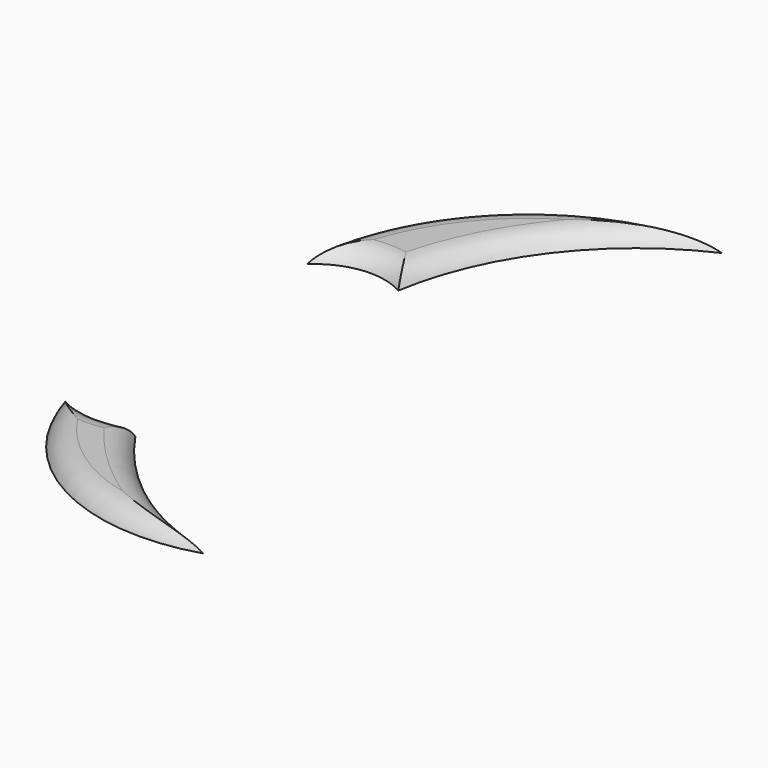
from build123d import *

# Parameters (mm, degrees)
F4_DEPTH      = 3
F5_T2_ANGLE   = 62.2477049864
F5_T4_ANGLE   = 129.1340791789
F5_T6_ANGLE   = 126.4050370347
F5_2_T2_ANGLE = 80.8778277447
F5_2_T4_ANGLE = 111.257856834
F5_2_T6_ANGLE = 169.7853810378


# Not quite as in the source:
# - a fillet or chamfer that OpenCascade refuses, or shapes differently, is made with other operations: its cross-section is extruded or revolved along the edge and cut away or added
# - a feature of the source that left no trace in its solid (it failed there, or was rolled back) is left out
# - the program builds the solid bodies; features that only make, move or delete a surface that nothing else refers to are left out


with BuildPart() as f4:
    # F3 (on Top) → F4 (new body)
    with BuildSketch(Plane.XY):
        with BuildLine():
            ThreePointArc((-5.3077070042, -31.2650799751), (-13.2021361292, -31.9649934775), (-20.5774232745, -29.0637817234))
            ThreePointArc((-20.5774232745, -29.0637817234), (-2.4043363453, -51.7875856508), (26.5503625851, -54.6612180769))
            ThreePointArc((26.5503625851, -54.6612180769), (8.5747716437, -45.7499050222), (-5.3077070042, -31.2650799751))
        make_face()
    extrude(amount=F4_DEPTH)

    # F5: fillet of radius 5 on 3 edges, made by hand

    # F5_s1 → F5_t2 (revolve, cut)
    with BuildSketch(Plane(origin=(42.5768459914, -3.8517260252, 0), x_dir=(0, 0, 1), z_dir=(0.9959329635, -0.0900973481, 0))):
        with BuildLine():
            ThreePointArc((0, 53.1706891683), (2.1833001327, 55.0146520758), (3, 57.7532648633))
            Line((3, 57.7532648633), (3, 53.1706891683))
            Line((3, 53.1706891683), (0, 53.1706891683))
        make_face()
    revolve(axis=Axis((43.0309999283, 1.1684758534, 3), (0, 0, -1)), revolution_arc=F5_T2_ANGLE, mode=Mode.SUBTRACT)

    # F5_s3 → F5_t4 (revolve, cut)
    with BuildSketch(Plane(origin=(-10.1562466974, -15.2654101251, 0), x_dir=(0, 0, 1), z_dir=(0.5539186056, 0.8325708248, 0))):
        with BuildLine():
            ThreePointArc((0, 16.5640855704), (2.1833001327, 18.4080484779), (3, 21.1466612654))
            Line((3, 21.1466612654), (3, 16.5640855704))
            Line((3, 16.5640855704), (0, 16.5640855704))
        make_face()
    revolve(axis=Axis((-10.7388300445, -14.8778109616, 3), (0, 0, -1)), revolution_arc=F5_T4_ANGLE, mode=Mode.SUBTRACT)

    # F5_s5 → F5_t6 (revolve, cut)
    with BuildSketch(Plane(origin=(-0.548879568, -18.3736765408, 0), x_dir=(0, 0, 1), z_dir=(0.029859828, 0.9995540959, 0))):
        with BuildLine():
            ThreePointArc((0, -21.4392018096), (2.1833001327, -19.5952389021), (3, -16.8566261146))
            Line((3, -16.8566261146), (3, -21.4392018096))
            Line((3, -21.4392018096), (0, -21.4392018096))
        make_face()
    revolve(axis=Axis((15.4842666098, -18.8526370977, 3), (0, 0, 1)), revolution_arc=F5_T6_ANGLE, mode=Mode.SUBTRACT)


with BuildPart() as f4b:
    # F3 (on Top) → F4, piece 2 (new body)
    with BuildSketch(Plane.XY):
        with BuildLine():
            ThreePointArc((-4.1721854359, 30.9002492577), (6.0474831917, 54.8040980412), (26.3369232416, 71.057535708))
            ThreePointArc((26.3369232416, 71.057535708), (-4.9982200607, 58.9572788508), (-20.3394051641, 29.0749184787))
            ThreePointArc((-20.3394051641, 29.0749184787), (-12.5583392109, 32.6672592136), (-4.1721854359, 30.9002492577))
        make_face()
    extrude(amount=F4_DEPTH)

    # F5#2: fillet of radius 5 on 3 edges, made by hand

    # F5_2_s1 → F5_2_t2 (revolve, cut)
    with BuildSketch(Plane(origin=(-1.1051572436, 19.683889291, 0), x_dir=(0, 0, 1), z_dir=(0.0560569838, -0.998427571, 0))):
        with BuildLine():
            ThreePointArc((0, 3.6571197259), (2.1833001327, 5.5010826334), (3, 8.2396954209))
            Line((3, 8.2396954209), (3, 3.6571197259))
            Line((3, 3.6571197259), (0, 3.6571197259))
        make_face()
    revolve(axis=Axis((48.6007815653, 22.4746425569, 3), (0, 0, -1)), revolution_arc=F5_2_T2_ANGLE, mode=Mode.SUBTRACT)

    # F5_2_s3 → F5_2_t4 (revolve, cut)
    with BuildSketch(Plane(origin=(19.5896273479, -4.7607351825, 0), x_dir=(0, 0, 1), z_dir=(0.9717166727, -0.2361497577, 0))):
        with BuildLine():
            ThreePointArc((0, -76.6524312792), (2.1833001327, -74.8084683718), (3, -72.0698555843))
            Line((3, -72.0698555843), (3, -76.6524312792))
            Line((3, -76.6524312792), (0, -76.6524312792))
        make_face()
    revolve(axis=Axis((26.5503625851, 23.8815236574, 3), (0, 0, 1)), revolution_arc=F5_2_T4_ANGLE, mode=Mode.SUBTRACT)

    # F5_2_s5 → F5_2_t6 (revolve, cut)
    with BuildSketch(Plane(origin=(-0.4514250872, 19.3811668147, 0), x_dir=(0, 0, 1), z_dir=(0.0232856303, -0.999728853, 0))):
        with BuildLine():
            ThreePointArc((0, 24.2003972309), (2.1833001327, 26.0443601383), (3, 28.7829729258))
            Line((3, 28.7829729258), (3, 24.2003972309))
            Line((3, 24.2003972309), (0, 24.2003972309))
        make_face()
    revolve(axis=Axis((-11.0304768119, 19.1347601151, 3), (0, 0, -1)), revolution_arc=F5_2_T6_ANGLE, mode=Mode.SUBTRACT)


solid = Compound([f4.part, f4b.part])
